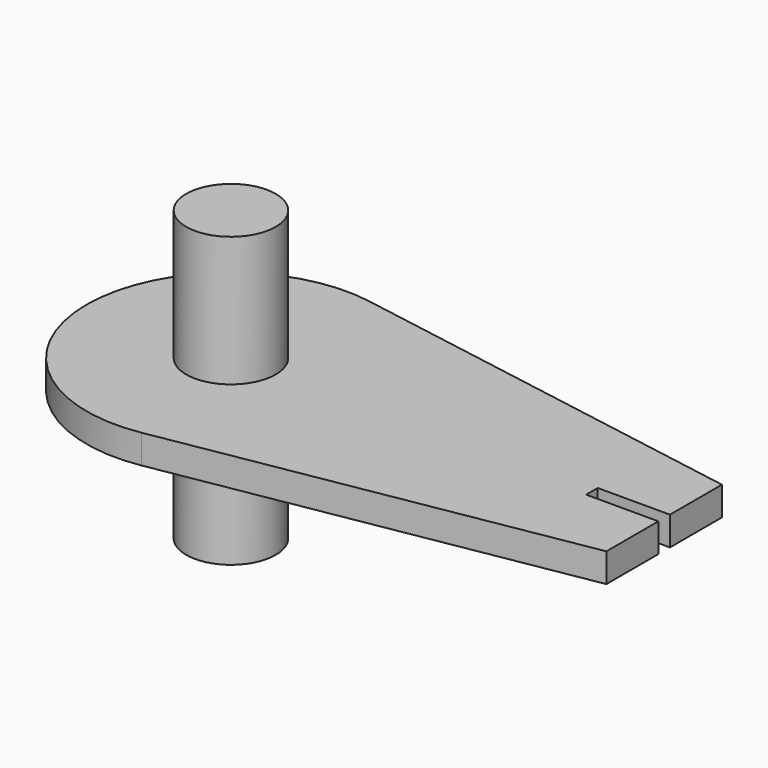
from build123d import *

# Parameters (mm, degrees)
F0_R     = 3.1
F1_DEPTH = 10
F2_DEPTH = 1
F3_W     = 5
F3_H     = 1
F4_DEPTH = 11.001


# Not quite as in the source:
# - a feature names something its author has since deleted; it is built from what else it names


with BuildPart() as f1:
    # F0 (on Top) → F1 (new body, symmetric)
    with BuildSketch(Plane.XY):
        Circle(F0_R)
    extrude(amount=F1_DEPTH, both=True)

    # F0 (on Top) → F2 (join, symmetric)
    with BuildSketch(Plane.XY):
        with BuildLine():
            ThreePointArc((1.6906573106, -9.8560477808), (7.645474907, -6.4456740103), (10, 0))
            ThreePointArc((10, 0), (7.6454749578, 6.44567395), (1.6906574661, 9.8560477542))
            ThreePointArc((1.6906574661, 9.8560477542), (-10, 7.89e-08), (1.6906573106, -9.8560477808))
        make_face()
        Circle(F0_R, mode=Mode.SUBTRACT)
        with BuildLine():
            ThreePointArc((1.6906574661, 9.8560477542), (7.6454749578, 6.44567395), (10, 0))
            ThreePointArc((10, 0), (7.645474907, -6.4456740103), (1.6906573106, -9.8560477808))
            Line((1.6906573106, -9.8560477808), (30, -5))
            Line((30, -5), (30, 5))
            Line((30, 5), (1.6906574661, 9.8560477542))
        make_face()
    extrude(amount=F2_DEPTH, both=True)

    # F3 (on face) → F4 (cut, through all)
    with BuildSketch(Plane.XY.offset(1)):
        with Locations((27.5, 0)):
            Rectangle(F3_W, F3_H)
    extrude(amount=-F4_DEPTH, mode=Mode.SUBTRACT)


solid = f1.part
